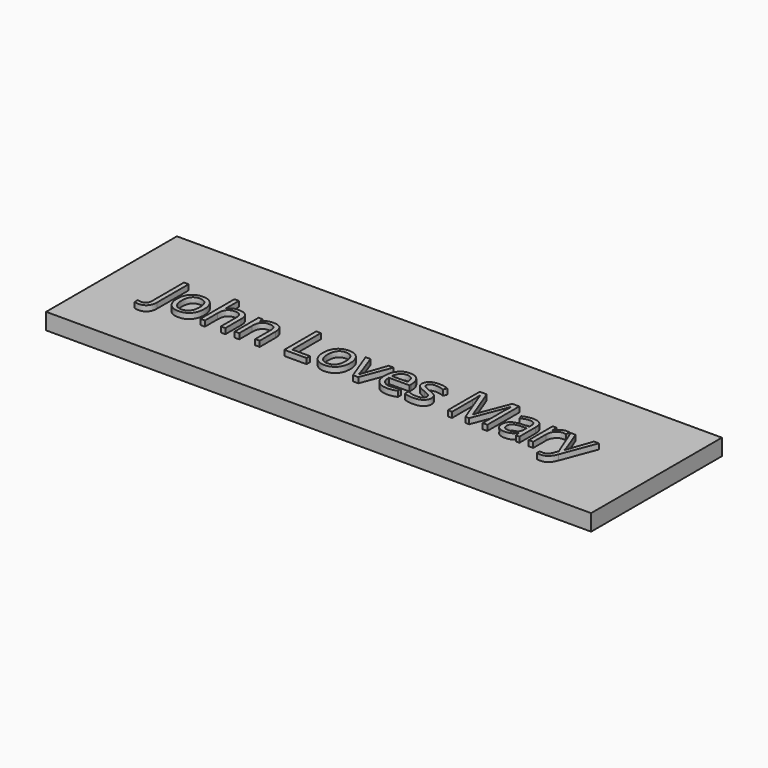
from build123d import *

# Parameters (mm, degrees)
F0_W         = 100
F0_H         = 30
F1_DEPTH     = 3
F2_TEXT_SIZE = 10.264840915
F3_DEPTH     = 1


# Not quite as in the source:
# - Text() gives the source's letters only with a copy of the font that has no kerning and outlines rounded to 1/6400 em; it was checked with that copy


with BuildPart() as f1:
    # F0 (on Top) → F1 (new body)
    with BuildSketch(Plane.XY):
        Rectangle(F0_W, F0_H)
    extrude(amount=F1_DEPTH)

    # F2 (on face) → F3 (join)
    with BuildSketch(Plane.XY.offset(3)):
        with Locations((-40, -4.3906854588)):
            Text('John Loves Mary', F2_TEXT_SIZE, font='Open Sans', text_align=(TextAlign.LEFT, TextAlign.BOTTOM))
    extrude(amount=F3_DEPTH)


solid = f1.part
